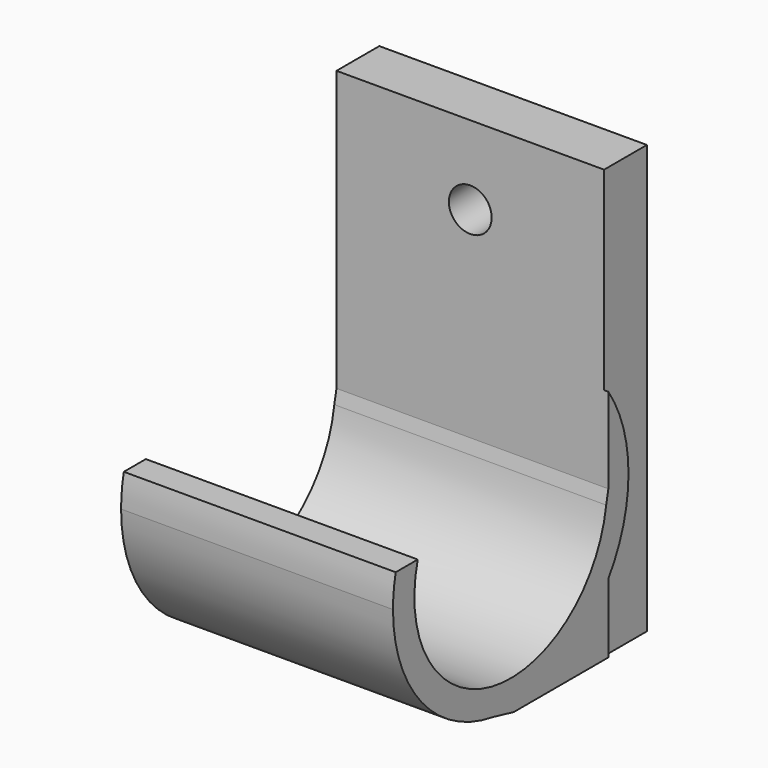
from build123d import *

# Parameters (mm, degrees)
F0_W      = 25
F0_H      = 40
F1_DEPTH  = 5
F6_DEPTH  = 25.4
F3_R      = 13.75
F7_DEPTH  = 25.4
F9_DEPTH  = 25.4
F2_R      = 11.25
F10_DEPTH = 25.4
F12_DEPTH = 25.4
F13_R     = 2
F14_DEPTH = 25.4


# Not quite as in the source:
# - a feature names something its author has since deleted; it is built from what else it names


with BuildPart() as f1:
    # F0 (on Front) → F1 (new body)
    with BuildSketch(Plane.XZ):
        Rectangle(F0_W, F0_H)
    extrude(amount=F1_DEPTH)

    # F3 (on face) → F6 (join)
    with BuildSketch(Plane(origin=(-12.5, 0, 0), x_dir=(0, -1, 0), z_dir=(-1, 0, 0))):
        with BuildLine():
            ThreePointArc((5, -13.5062897776), (20.4196296212, -18.9696149078), (30.1510077715, -5.8199693449))
            ThreePointArc((30.1510077715, -5.8199693449), (20.4196296212, 7.329676218), (5, 1.8663510878))
            Line((5, 1.8663510878), (5, -13.5062897776))
        make_face()
    extrude(amount=-F6_DEPTH)

    # F3 (on face) → F7 (join)
    with BuildSketch(Plane(origin=(-12.5, 0, 0), x_dir=(0, -1, 0), z_dir=(-1, 0, 0))):
        with Locations((16.4010077715, -5.8199693449)):
            Circle(F3_R)
    extrude(amount=-F7_DEPTH)

    # F8 (on face) → F9 (join)
    with BuildSketch(Plane(origin=(-12.5, 0, 0), x_dir=(0, -1, 0), z_dir=(-1, 0, 0))):
        Polygon((5, -12.7877519428), (5, -19.9861098081), (16.0521287471, -19.9861098081), (19.5415690541, -19.1552899778), (7.0377378725, -15.2296693996), align=None)
    extrude(amount=-F9_DEPTH)

    # F2 (on face) → F10 (cut)
    with BuildSketch(Plane(origin=(-12.5, 0, 0), x_dir=(0, -1, 0), z_dir=(-1, 0, 0))):
        with Locations((16.4017565548, -5.8220350184)):
            Circle(F2_R)
    extrude(amount=-F10_DEPTH, mode=Mode.SUBTRACT)

    # F11 (on face) → F12 (cut)
    with BuildSketch(Plane(origin=(-12.5, 0, 0), x_dir=(0, -1, 0), z_dir=(-1, 0, 0))):
        Polygon((12.1690463275, 13.4603166953), (5, 3.5622220363), (5, -6.1200439696), (5.3498325869, -7.8012463637), (19.8114402592, -7.8012463637), (20.6344667822, -2.8826519847), (33.6853265762, -2.8826519847), (32.509572804, 10.7560846955), align=None)
    extrude(amount=-F12_DEPTH, mode=Mode.SUBTRACT)

    # F13 (on face) → F14 (cut)
    with BuildSketch(Plane.XZ.offset(5)):
        with Locations((0, 12.6415221021)):
            Circle(F13_R)
    extrude(amount=-F14_DEPTH, mode=Mode.SUBTRACT)


solid = f1.part
